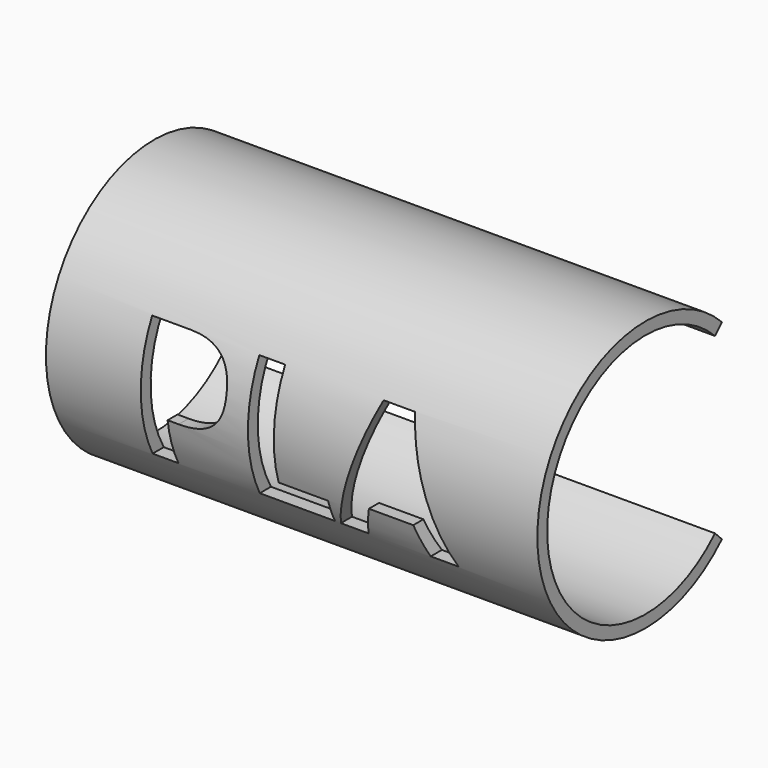
from build123d import *

# Parameters (mm, degrees)
F1_DEPTH     = 50.8
F3_TEXT_SIZE = 17.6388888889
F4_DEPTH     = 35.2792817332


# Not quite as in the source:
# - Text() gives the source's letters only with a copy of the font that has no kerning and outlines rounded to 1/6400 em; it was checked with that copy


with BuildPart() as f1:
    # F0 (on Right) → F1 (new body)
    with BuildSketch(Plane.YZ):
        with BuildLine():
            ThreePointArc((8.9802561211, -8.9802561211), (-12.7, 0), (8.9802561211, 8.9802561211))
            Line((8.9802561211, 8.9802561211), (9.8782817332, 9.8782817332))
            ThreePointArc((9.8782817332, 9.8782817332), (-13.97, 0), (9.8782817332, -9.8782817332))
            Line((9.8782817332, -9.8782817332), (8.9802561211, -8.9802561211))
        make_face()
    extrude(amount=F1_DEPTH)

    # F3 (on offset) → F4 (cut, through all)
    with BuildSketch(Plane.XZ.offset(25.4)):
        with Locations((8.2213758681, -6.35)):
            Text('PLA', F3_TEXT_SIZE, font='Open Sans', font_style=FontStyle.BOLD, text_align=(TextAlign.LEFT, TextAlign.BOTTOM))
        with BuildLine():
            Line((12.4767578125, 4.0541883681), (12.4767578125, 0.3169487847))
            Line((12.4767578125, 0.3169487847), (13.3559461806, 0.3169487847))
            add(Edge.make_bspline(
                [(13.3559461806, 0.3169487847), (14.58515625, 0.3169487847), (15.1970052083, 0.8033962674)],
                knots=[0, 0, 0, 1, 1, 1], degree=2))
            add(Edge.make_bspline(
                [(15.1970052083, 0.8033962674), (15.8088541667, 1.28984375), (15.8088541667, 2.2186414931)],
                knots=[0, 0, 0, 1, 1, 1], degree=2))
            add(Edge.make_bspline(
                [(15.8088541667, 2.2186414931), (15.8088541667, 3.1584635417), (15.2962239583, 3.6063259549)],
                knots=[0, 0, 0, 1, 1, 1], degree=2))
            add(Edge.make_bspline(
                [(15.2962239583, 3.6063259549), (14.78359375, 4.0541883681), (13.6894314236, 4.0541883681)],
                knots=[0, 0, 0, 1, 1, 1], degree=2))
            Line((13.6894314236, 4.0541883681), (12.4767578125, 4.0541883681))
        make_face()
        with BuildLine():
            Line((33.7261067708, -1.1134548611), (37.0058376736, -1.1134548611))
            add(Edge.make_bspline(
                [(37.0058376736, -1.1134548611), (35.7407986111, 2.9600260417), (35.5809461806, 3.4947048611)],
                knots=[0, 0, 0, 1, 1, 1], degree=2))
            add(Edge.make_bspline(
                [(35.5809461806, 3.4947048611), (35.42109375, 4.0293836806), (35.3521918403, 4.3380642361)],
                knots=[0, 0, 0, 1, 1, 1], degree=2))
            add(Edge.make_bspline(
                [(35.3521918403, 4.3380642361), (35.0683159722, 3.2356336806), (33.7261067708, -1.1134548611)],
                knots=[0, 0, 0, 1, 1, 1], degree=2))
        make_face()
    extrude(amount=-F4_DEPTH, mode=Mode.SUBTRACT)


solid = f1.part
